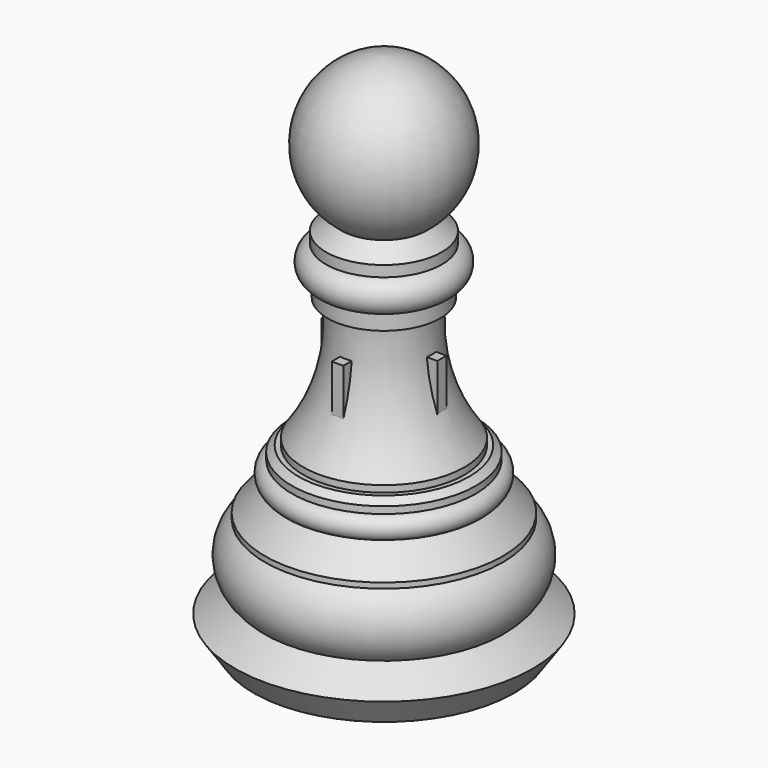
from build123d import *

# Parameters (mm, degrees)
F2_W            = 1.3378583826
F2_H            = 4.2365510017
F3_DEPTH        = 0.5
F3_COPIES_COUNT = 4


# Not quite as in the source:
# - a pattern or mirror of a feature is missing from the dataset's text; its kind, count and spacing are read off the source's solid


with BuildPart() as f1:
    # F0 (on Front) → F1 (revolve)
    with BuildSketch(Plane.XZ):
        with BuildLine():
            Line((0, 45), (0, 0))
            Line((0, 0), (11.2852290238, 0))
            Line((11.2852290238, 0), (12.9102486834, 2.3947660588))
            Line((12.9102486834, 2.3947660588), (10.3100675682, 4.1591744925))
            ThreePointArc((10.3100675682, 4.1591744925), (11.6004195133, 6.9094906196), (10.3100675682, 9.6598067467))
            Line((10.3100675682, 9.6598067467), (10.3100675682, 10.1309951941))
            Line((10.3100675682, 10.1309951941), (8.3843368541, 12.3686434379))
            ThreePointArc((8.3843368541, 12.3686434379), (8.7331630293, 13.3811939937), (7.9746896115, 14.1372736211))
            Line((7.9746896115, 14.1372736211), (7.9746896115, 14.7359652811))
            Line((7.9746896115, 14.7359652811), (7.3973798121, 15.2491294988))
            Line((7.3973798121, 15.2491294988), (6.980433749, 15.2491294988))
            Line((6.980433749, 15.2491294988), (6.980433749, 15.8264392982))
            ThreePointArc((6.980433749, 15.8264392982), (4.6239411518, 20.7485026373), (4.180635733, 26.1875508242))
            Line((4.180635733, 26.1875508242), (4.8862364052, 26.5082782969))
            Line((4.8862364052, 26.5082782969), (4.8862364052, 27.8553350765))
            ThreePointArc((4.8862364052, 27.8553350765), (6.052835472, 29.2053516541), (5.0145278591, 30.6563566312))
            Line((5.0145278591, 30.6563566312), (5.0145278591, 31.5971579148))
            Line((5.0145278591, 31.5971579148), (3.6674716605, 32.7945409442))
            ThreePointArc((3.6674716605, 32.7945409442), (6.1332426057, 40.1891775754), (0, 45))
        make_face()
    revolve(axis=Axis((0, 0, 22.5), (0, 0, -1)))

    # F2 (on Front) → F3 (join, symmetric)
    with BuildSketch(Plane.XZ):
        with Locations((4.3546957895, 21.3884068653)):
            Rectangle(F2_W, F2_H)
    f3 = extrude(amount=F3_DEPTH, both=True)

    # F3_copies: F3 ×4 about axis
    f3_copies_axis = Axis((0, 0, 0), (0, 0, 1))
    for i in range(1, F3_COPIES_COUNT):
        add(f3.rotate(f3_copies_axis, i * 360 / F3_COPIES_COUNT))


solid = f1.part
